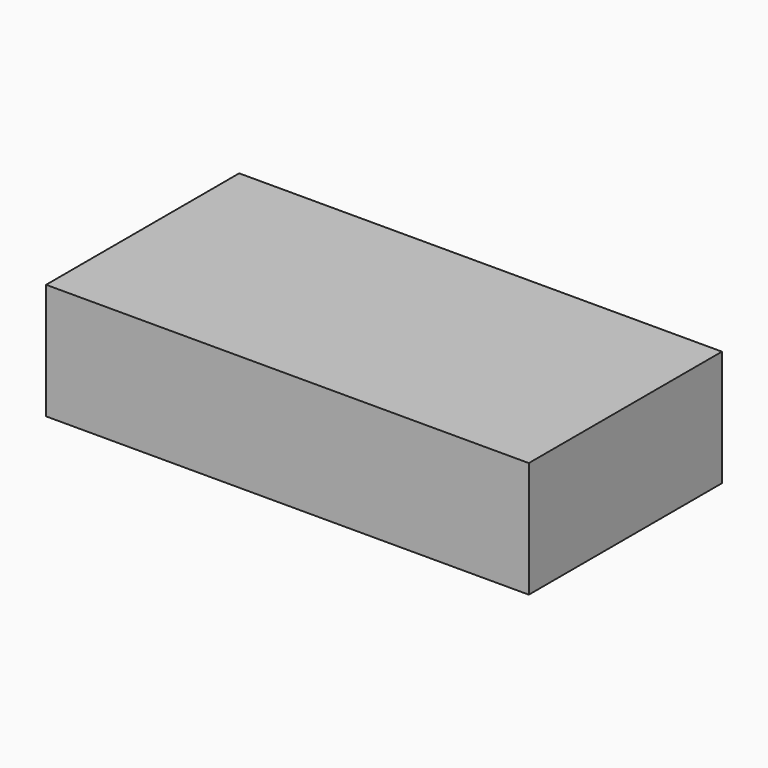
from build123d import *

# Parameters (mm, degrees)
F0_W     = 50
F0_H     = 12
F1_DEPTH = 12.5


# Not quite as in the source:
# - a feature of the source that left no trace in its solid (it failed there, or was rolled back) is left out


with BuildPart() as f1:
    # F0 (on Front) → F1 (new body, symmetric)
    with BuildSketch(Plane.XZ):
        with Locations((25, 6)):
            Rectangle(F0_W, F0_H)
    extrude(amount=F1_DEPTH, both=True)


solid = f1.part
